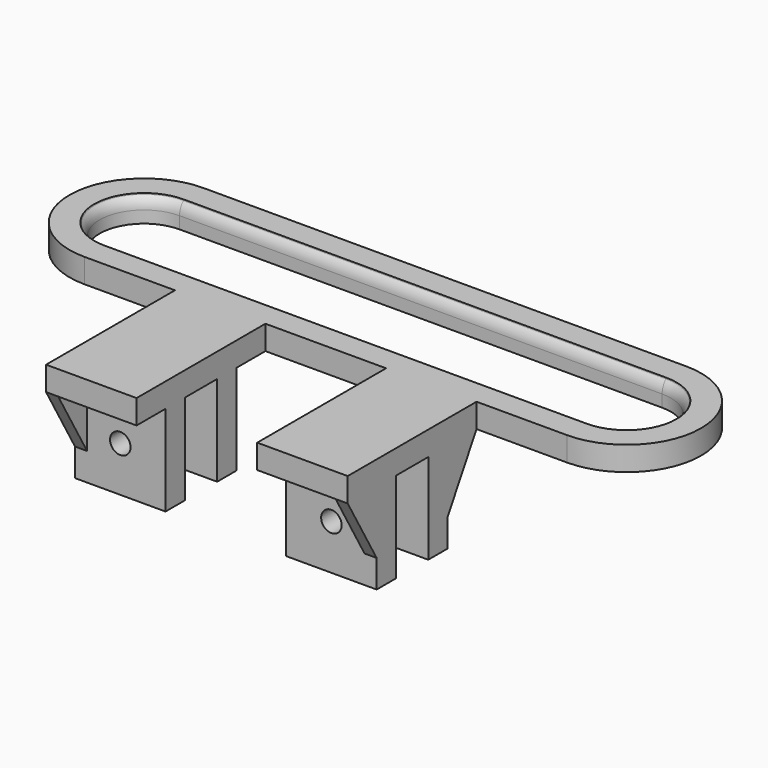
from build123d import *

# Parameters (mm, degrees)
F3_W      = 15
F3_H      = 4
F4_DEPTH  = 26.7
F5_W      = 15
F5_H      = 4
F6_DEPTH  = 15
F7_R      = 1.7
F8_DEPTH  = 45.4048897462
F10_DEPTH = 2
F12_DEPTH = 2


with BuildPart() as f2:
    # F2: sweep along a path in F0
    with BuildLine(Plane.XY) as f2_path:
        ThreePointArc((-40, 26.8490467115), (-50, 16.8490467115), (-40, 6.8490467115))
        Line((-40, 6.8490467115), (40, 6.8490467115))
        ThreePointArc((40, 6.8490467115), (50, 16.8490467115), (40, 26.8490467115))
        Line((40, 26.8490467115), (-40, 26.8490467115))
    # F1 (on Right) → F2 (sweep)
    with BuildSketch(Plane.YZ):
        with BuildLine():
            Line((4.4971018384, 2), (4.4971018384, -2))
            Line((4.4971018384, -2), (9.4971018384, -2))
            Line((9.4971018384, -2), (9.4971018384, 0))
            ThreePointArc((9.4971018384, 0), (9.2955306442, 1.013366825), (8.7215044486, 1.8724577372))
            Line((8.7215044486, 1.8724577372), (8.5939621858, 2))
            Line((8.5939621858, 2), (4.4971018384, 2))
        make_face()
    sweep(path=f2_path.line)

    # F3 (on face) → F4 (join)
    with BuildSketch(Plane.XZ.offset(-4.4971018384)):
        with Locations((-17.5, 0)):
            Rectangle(F3_W, F3_H)
        with Locations((17.5, 0)):
            Rectangle(F3_W, F3_H)
    extrude(amount=F4_DEPTH)

    # F5 (on face) → F6 (join)
    with BuildSketch(Plane(origin=(0, 0, -2), x_dir=(1, 0, 0), z_dir=(0, 0, -1))):
        with Locations((-17.5, 14.2028981616)):
            Rectangle(F5_W, F5_H)
        with Locations((-17.5, 3.5028981616)):
            Rectangle(F5_W, F5_H)
        with Locations((17.5, 14.2028981616)):
            Rectangle(F5_W, F5_H)
        with Locations((17.5, 3.5028981616)):
            Rectangle(F5_W, F5_H)
    extrude(amount=F6_DEPTH)

    # F7 (on face) → F8 (cut, through all)
    with BuildSketch(Plane.XZ.offset(16.2028981616)):
        with Locations((-17.5, -9.5)):
            Circle(F7_R)
        with Locations((17.5, -9.5)):
            Circle(F7_R)
    extrude(amount=-F8_DEPTH, mode=Mode.SUBTRACT)

    # F9 (on face) → F10 (join)
    with BuildSketch(Plane(origin=(-25, 0, 0), x_dir=(0, -1, 0), z_dir=(-1, 0, 0))):
        Polygon((1.5028981616, -12.3923048454), (1.5028981616, -2), (-4.4971018384, -2), align=None)
        Polygon((22.2028981616, -2), (16.2028981616, -2), (16.2028981616, -12.3923048454), align=None)
    extrude(amount=-F10_DEPTH)

    # F11 (on face) → F12 (join)
    with BuildSketch(Plane.YZ.offset(25)):
        Polygon((-16.2028981616, -12.3923048454), (-16.2028981616, -2), (-22.2028981616, -2), align=None)
        Polygon((-1.5028981616, -12.3923048454), (4.4971018384, -2), (-1.5028981616, -2), align=None)
    extrude(amount=-F12_DEPTH)


solid = f2.part
